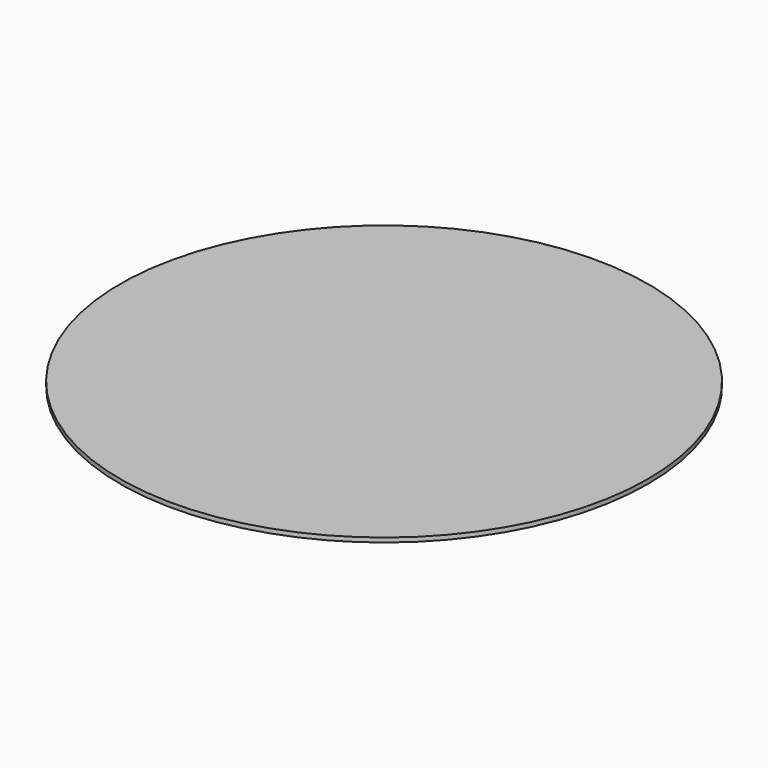
from build123d import *

# Parameters (mm, degrees)
F0_R     = 59.8781505206
F1_DEPTH = 1


# Not quite as in the source:
# - the program builds the solid bodies; features that only make, move or delete a surface that nothing else refers to are left out


with BuildPart() as f1:
    # F0 (on Top) → F1 (new body)
    with BuildSketch(Plane.XY):
        Circle(F0_R)
    extrude(amount=F1_DEPTH)


solid = f1.part
